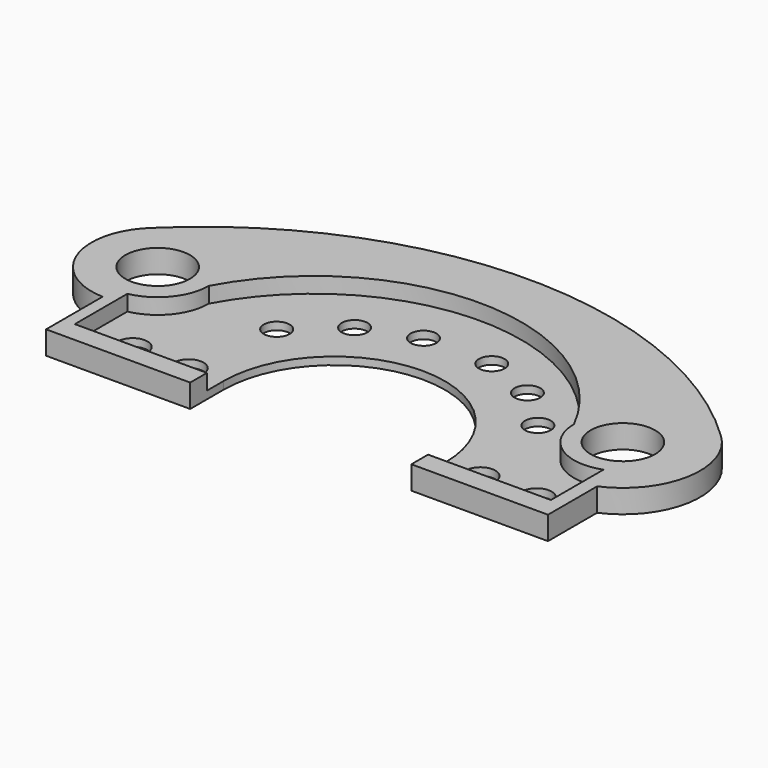
from build123d import *

# Parameters (mm, degrees)
F0_R     = 3.9142983579
F0_R_2   = 3.3882320549
F0_R_3   = 3.3768548991
F1_DEPTH = 2
F0_R_4   = 8.4535282778
F0_R_5   = 8.4613165319
F5_DEPTH = 6
F6_DEPTH = 6
F7_DEPTH = 6.096


# Not quite as in the source:
# - the program builds the solid bodies; features that only make, move or delete a surface that nothing else refers to are left out


with BuildPart() as f1:
    # F0 (on Top) → F1 (new body)
    with BuildSketch(Plane.XY):
        with BuildLine():
            Line((-5.016844254, 60.8599856496), (-5.016844254, 55.3855970502))
            Line((-5.016844254, 55.3855970502), (27.1643232554, 55.3855970502))
            Line((27.1643232554, 55.3855970502), (27.1643232554, 72.5930482149))
            ThreePointArc((27.1643232554, 72.5930482149), (15.3743446714, 74.0537278173), (9.8619121261, 84.5775231091))
            ThreePointArc((9.8619121261, 84.5775231091), (-38.0783668351, 114.5002429814), (-86.734496244, 85.7561899899))
            ThreePointArc((-86.734496244, 85.7561899899), (-89.789886214, 77.2334083533), (-97.5642204285, 72.5930482149))
            Line((-97.5642204285, 72.5930482149), (-97.5642204285, 55.3855970502))
            Line((-97.5642204285, 55.3855970502), (-82.5288370252, 55.3855970502))
            Line((-82.5288370252, 55.3855970502), (-62.9575885832, 55.3855970502))
            Line((-62.9575885832, 55.3855970502), (-62.9575885832, 60.8599856496))
            ThreePointArc((-62.9575885832, 60.8599856496), (-33.9872164186, 89.8303578142), (-5.016844254, 60.8599856496))
        make_face()
        with Locations((-86.9268402457, 61.0230416059)):
            Circle(F0_R, mode=Mode.SUBTRACT)
        with Locations((-72.1179321408, 60.8599856496)):
            Circle(F0_R, mode=Mode.SUBTRACT)
        with Locations((-68.8042789698, 85.551418364)):
            Circle(F0_R_2, mode=Mode.SUBTRACT)
        with Locations((4.3670018204, 60.8045533299)):
            Circle(F0_R, mode=Mode.SUBTRACT)
        with Locations((19.1759099253, 60.7153773308)):
            Circle(F0_R, mode=Mode.SUBTRACT)
        with Locations((-0.4634411598, 85.6597200036)):
            Circle(F0_R_3, mode=Mode.SUBTRACT)
        with Locations((-56.8258166313, 96.0706025362)):
            Circle(F0_R_3, mode=Mode.SUBTRACT)
        with Locations((-42.8707525134, 101.2179628015)):
            Circle(F0_R_3, mode=Mode.SUBTRACT)
        with Locations((-11.1492751166, 95.5843403935)):
            Circle(F0_R_3, mode=Mode.SUBTRACT)
        with Locations((-24.9121841043, 101.1035814881)):
            Circle(F0_R_3, mode=Mode.SUBTRACT)
    extrude(amount=F1_DEPTH)

    # F0 (on Top) → F5 (join)
    with BuildSketch(Plane.XY):
        with BuildLine():
            ThreePointArc((30.7714908133, 66.0106175583), (42.611434574, 81.0345848644), (36.6692617536, 99.2168411613))
            ThreePointArc((36.6692617536, 99.2168411613), (-37.7049289316, 128.8806796099), (-111.8238263521, 98.5845974088))
            ThreePointArc((-111.8238263521, 98.5845974088), (-116.4247817384, 79.7587957054), (-100.7084514224, 68.4196351703))
            Line((-100.7084514224, 68.4196351703), (-100.7084514224, 49.9112084508))
            Line((-100.7084514224, 49.9112084508), (-62.9575885832, 49.9112084508))
            Line((-62.9575885832, 49.9112084508), (-62.9575885832, 55.3855970502))
            Line((-62.9575885832, 55.3855970502), (-82.5288370252, 55.3855970502))
            Line((-82.5288370252, 55.3855970502), (-97.5642204285, 55.3855970502))
            Line((-97.5642204285, 55.3855970502), (-97.5642204285, 72.5930482149))
            ThreePointArc((-97.5642204285, 72.5930482149), (-89.789886214, 77.2334083533), (-86.734496244, 85.7561899899))
            ThreePointArc((-86.734496244, 85.7561899899), (-38.0783668351, 114.5002429814), (9.8619121261, 84.5775231091))
            ThreePointArc((9.8619121261, 84.5775231091), (15.3743446714, 74.0537278173), (27.1643232554, 72.5930482149))
            Line((27.1643232554, 72.5930482149), (27.1643232554, 55.3855970502))
            Line((27.1643232554, 55.3855970502), (-5.016844254, 55.3855970502))
            Line((-5.016844254, 55.3855970502), (-5.016844254, 49.9112084508))
            Line((-5.016844254, 49.9112084508), (30.7714908133, 49.9112084508))
            Line((30.7714908133, 49.9112084508), (30.7714908133, 66.0106175583))
        make_face()
        with Locations((-100.1490219674, 85.7561899899)):
            Circle(F0_R_4, mode=Mode.SUBTRACT)
        with Locations((22.6636270451, 84.5775231091)):
            Circle(F0_R_5, mode=Mode.SUBTRACT)
    extrude(amount=F5_DEPTH)

    # F0 (on Top) → F6 (join)
    with BuildSketch(Plane.XY):
        with BuildLine():
            ThreePointArc((30.7714908133, 66.0106175583), (42.611434574, 81.0345848644), (36.6692617536, 99.2168411613))
            ThreePointArc((36.6692617536, 99.2168411613), (-37.7049289316, 128.8806796099), (-111.8238263521, 98.5845974088))
            ThreePointArc((-111.8238263521, 98.5845974088), (-116.4247817384, 79.7587957054), (-100.7084514224, 68.4196351703))
            Line((-100.7084514224, 68.4196351703), (-100.7084514224, 49.9112084508))
            Line((-100.7084514224, 49.9112084508), (-62.9575885832, 49.9112084508))
            Line((-62.9575885832, 49.9112084508), (-62.9575885832, 55.3855970502))
            Line((-62.9575885832, 55.3855970502), (-82.5288370252, 55.3855970502))
            Line((-82.5288370252, 55.3855970502), (-97.5642204285, 55.3855970502))
            Line((-97.5642204285, 55.3855970502), (-97.5642204285, 72.5930482149))
            ThreePointArc((-97.5642204285, 72.5930482149), (-89.789886214, 77.2334083533), (-86.734496244, 85.7561899899))
            ThreePointArc((-86.734496244, 85.7561899899), (-38.0783668351, 114.5002429814), (9.8619121261, 84.5775231091))
            ThreePointArc((9.8619121261, 84.5775231091), (15.3743446714, 74.0537278173), (27.1643232554, 72.5930482149))
            Line((27.1643232554, 72.5930482149), (27.1643232554, 55.3855970502))
            Line((27.1643232554, 55.3855970502), (-5.016844254, 55.3855970502))
            Line((-5.016844254, 55.3855970502), (-5.016844254, 49.9112084508))
            Line((-5.016844254, 49.9112084508), (30.7714908133, 49.9112084508))
            Line((30.7714908133, 49.9112084508), (30.7714908133, 66.0106175583))
        make_face()
        with Locations((-100.1490219674, 85.7561899899)):
            Circle(F0_R_4, mode=Mode.SUBTRACT)
        with Locations((22.6636270451, 84.5775231091)):
            Circle(F0_R_5, mode=Mode.SUBTRACT)
    extrude(amount=F6_DEPTH)

    # F0 (on Top) → F7 (join)
    with BuildSketch(Plane.XY):
        with BuildLine():
            ThreePointArc((30.7714908133, 66.0106175583), (42.611434574, 81.0345848644), (36.6692617536, 99.2168411613))
            ThreePointArc((36.6692617536, 99.2168411613), (-37.7049289316, 128.8806796099), (-111.8238263521, 98.5845974088))
            ThreePointArc((-111.8238263521, 98.5845974088), (-116.4247817384, 79.7587957054), (-100.7084514224, 68.4196351703))
            Line((-100.7084514224, 68.4196351703), (-100.7084514224, 49.9112084508))
            Line((-100.7084514224, 49.9112084508), (-62.9575885832, 49.9112084508))
            Line((-62.9575885832, 49.9112084508), (-62.9575885832, 55.3855970502))
            Line((-62.9575885832, 55.3855970502), (-82.5288370252, 55.3855970502))
            Line((-82.5288370252, 55.3855970502), (-97.5642204285, 55.3855970502))
            Line((-97.5642204285, 55.3855970502), (-97.5642204285, 72.5930482149))
            ThreePointArc((-97.5642204285, 72.5930482149), (-89.789886214, 77.2334083533), (-86.734496244, 85.7561899899))
            ThreePointArc((-86.734496244, 85.7561899899), (-38.0783668351, 114.5002429814), (9.8619121261, 84.5775231091))
            ThreePointArc((9.8619121261, 84.5775231091), (15.3743446714, 74.0537278173), (27.1643232554, 72.5930482149))
            Line((27.1643232554, 72.5930482149), (27.1643232554, 55.3855970502))
            Line((27.1643232554, 55.3855970502), (-5.016844254, 55.3855970502))
            Line((-5.016844254, 55.3855970502), (-5.016844254, 49.9112084508))
            Line((-5.016844254, 49.9112084508), (30.7714908133, 49.9112084508))
            Line((30.7714908133, 49.9112084508), (30.7714908133, 66.0106175583))
        make_face()
        with Locations((-100.1490219674, 85.7561899899)):
            Circle(F0_R_4, mode=Mode.SUBTRACT)
        with Locations((22.6636270451, 84.5775231091)):
            Circle(F0_R_5, mode=Mode.SUBTRACT)
    extrude(amount=F7_DEPTH)


solid = f1.part
